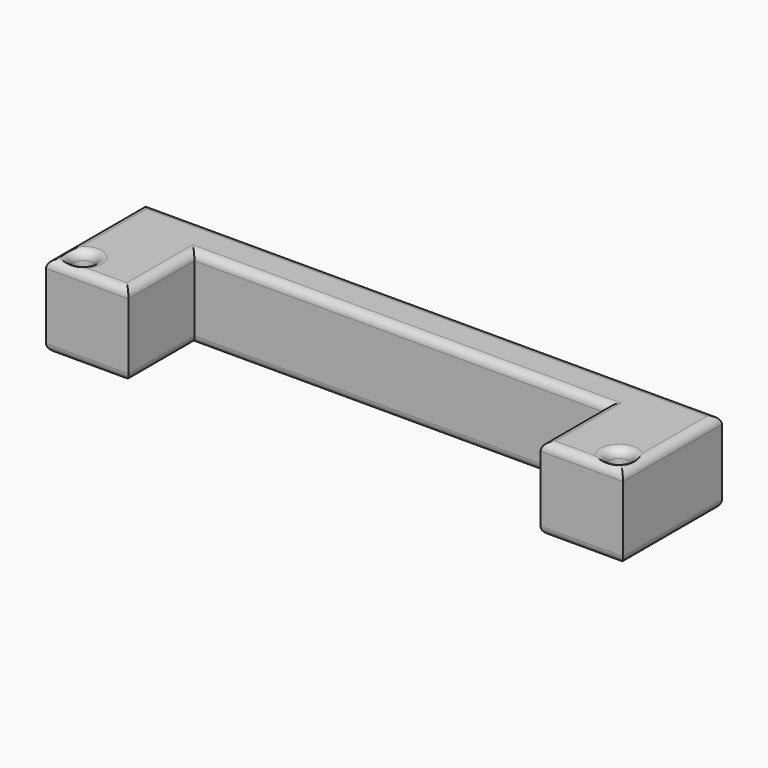
from build123d import *

# Parameters (mm, degrees)
F1_DEPTH     = 20
F3_D         = 5
F5_T1_DEPTH  = 150
F5_T3_DEPTH  = 40
F5_T5_DEPTH  = 30
F5_T7_DEPTH  = 25
F5_T9_DEPTH  = 100
F5_T11_DEPTH = 30
F5_T25_DEPTH = 105
F5_T29_DEPTH = 30
F5_T36_DEPTH = 30
F5_T40_DEPTH = 105
F5_T47_DEPTH = 30
F5_T51_DEPTH = 105
F5_T58_DEPTH = 105
F5_T62_DEPTH = 30


# Not quite as in the source:
# - a fillet or chamfer that OpenCascade refuses, or shapes differently, is made with other operations: its cross-section is extruded or revolved along the edge and cut away or added


with BuildPart() as f1:
    # F0 (on Top) → F1 (new body)
    with BuildSketch(Plane.XY):
        Polygon((70, 30), (0, 30), (0, 20), (50, 20), (50, 0), (70, 0), align=None)
    extrude(amount=F1_DEPTH)

    # F3 (through all)
    with Locations(Plane(origin=(0, 0, 0), x_dir=(1, 0, 0), z_dir=(0, 0, -1))):
        with Locations((65, -5)):
            Hole(F3_D / 2)

    # F4: F1 across plane


with BuildPart() as f1_1:
    add(f1.part)
    add(f1.part.mirror(Plane.YZ))

    # F5: fillet of radius 2 on 20 edges, made by hand

    # F5_s2 → F5_t1 (cut)
    with BuildSketch(Plane.YZ.offset(-75)):
        with BuildLine():
            ThreePointArc((30, 18), (29.4142135624, 19.4142135624), (28, 20))
            Line((28, 20), (30, 20))
            Line((30, 20), (30, 18))
        make_face()
        with BuildLine():
            ThreePointArc((30, 2), (29.4142135624, 0.5857864376), (28, 0))
            Line((28, 0), (30, 0))
            Line((30, 0), (30, 2))
        make_face()
    extrude(amount=F5_T1_DEPTH, mode=Mode.SUBTRACT)

    # F5_s4 → F5_t3 (cut)
    with BuildSketch(Plane.XZ.offset(-35)):
        with BuildLine():
            ThreePointArc((-70, 18), (-69.4142135624, 19.4142135624), (-68, 20))
            Line((-68, 20), (-70, 20))
            Line((-70, 20), (-70, 18))
        make_face()
        with BuildLine():
            ThreePointArc((68, 20), (69.4142135624, 19.4142135624), (70, 18))
            Line((70, 18), (70, 20))
            Line((70, 20), (68, 20))
        make_face()
        with BuildLine():
            ThreePointArc((-68, 0), (-69.4142135624, 0.5857864376), (-70, 2))
            Line((-70, 2), (-70, 0))
            Line((-70, 0), (-68, 0))
        make_face()
        with BuildLine():
            ThreePointArc((68, 0), (69.4142135624, 0.5857864376), (70, 2))
            Line((70, 2), (70, 0))
            Line((70, 0), (68, 0))
        make_face()
    extrude(amount=F5_T3_DEPTH, mode=Mode.SUBTRACT)

    # F5_s6 → F5_t5 (cut)
    with BuildSketch(Plane.YZ.offset(-75)):
        with BuildLine():
            ThreePointArc((0, 18), (0.5857864376, 19.4142135624), (2, 20))
            Line((2, 20), (0, 20))
            Line((0, 20), (0, 18))
        make_face()
        with BuildLine():
            ThreePointArc((2, 0), (0.5857864376, 0.5857864376), (0, 2))
            Line((0, 2), (0, 0))
            Line((0, 0), (2, 0))
        make_face()
    extrude(amount=F5_T5_DEPTH, mode=Mode.SUBTRACT)

    # F5_s8 → F5_t7 (cut)
    with BuildSketch(Plane.XZ.offset(-20)):
        with BuildLine():
            ThreePointArc((-50, 18), (-50.5857864376, 19.4142135624), (-52, 20))
            Line((-52, 20), (-50, 20))
            Line((-50, 20), (-50, 18))
        make_face()
        with BuildLine():
            ThreePointArc((50, 18), (50.5857864376, 19.4142135624), (52, 20))
            Line((52, 20), (50, 20))
            Line((50, 20), (50, 18))
        make_face()
        with BuildLine():
            ThreePointArc((-52, 0), (-50.5857864376, 0.5857864376), (-50, 2))
            Line((-50, 2), (-50, 0))
            Line((-50, 0), (-52, 0))
        make_face()
        with BuildLine():
            ThreePointArc((52, 0), (50.5857864376, 0.5857864376), (50, 2))
            Line((50, 2), (50, 0))
            Line((50, 0), (52, 0))
        make_face()
    extrude(amount=F5_T7_DEPTH, mode=Mode.SUBTRACT)

    # F5_s10 → F5_t9 (cut)
    with BuildSketch(Plane.YZ.offset(-50)):
        with BuildLine():
            ThreePointArc((20, 18), (20.5857864376, 19.4142135624), (22, 20))
            Line((22, 20), (20, 20))
            Line((20, 20), (20, 18))
        make_face()
        with BuildLine():
            ThreePointArc((22, 0), (20.5857864376, 0.5857864376), (20, 2))
            Line((20, 2), (20, 0))
            Line((20, 0), (22, 0))
        make_face()
    extrude(amount=F5_T9_DEPTH, mode=Mode.SUBTRACT)

    # F5_s12 → F5_t11 (cut)
    with BuildSketch(Plane.YZ.offset(45)):
        with BuildLine():
            ThreePointArc((0, 18), (0.5857864376, 19.4142135624), (2, 20))
            Line((2, 20), (0, 20))
            Line((0, 20), (0, 18))
        make_face()
        with BuildLine():
            ThreePointArc((2, 0), (0.5857864376, 0.5857864376), (0, 2))
            Line((0, 2), (0, 0))
            Line((0, 0), (2, 0))
        make_face()
    extrude(amount=F5_T11_DEPTH, mode=Mode.SUBTRACT)

    # F5_s13 → F5_t14 (revolve, cut)
    with BuildSketch(Plane.XZ.offset(-5)):
        with BuildLine():
            ThreePointArc((67.5, 18), (68.0857864376, 19.4142135624), (69.5, 20))
            Line((69.5, 20), (67.5, 20))
            Line((67.5, 20), (67.5, 18))
        make_face()
    revolve(axis=Axis((65, 5, 20), (0, 0, -1)), mode=Mode.SUBTRACT)

    # F5_s15 → F5_t16 (revolve, cut)
    with BuildSketch(Plane.XZ.offset(-5)):
        with BuildLine():
            ThreePointArc((-67.5, 18), (-68.0857864376, 19.4142135624), (-69.5, 20))
            Line((-69.5, 20), (-67.5, 20))
            Line((-67.5, 20), (-67.5, 18))
        make_face()
    revolve(axis=Axis((-65, 5, 20), (0, 0, 1)), mode=Mode.SUBTRACT)

    # F5_s17 → F5_t18 (revolve, cut)
    with BuildSketch(Plane.XZ.offset(-5)):
        with BuildLine():
            ThreePointArc((69.5, 0), (68.0857864376, 0.5857864376), (67.5, 2))
            Line((67.5, 2), (67.5, 0))
            Line((67.5, 0), (69.5, 0))
        make_face()
    revolve(axis=Axis((65, 5, 0), (0, 0, -1)), mode=Mode.SUBTRACT)

    # F5_s19 → F5_t20 (revolve, cut)
    with BuildSketch(Plane.XZ.offset(-5)):
        with BuildLine():
            ThreePointArc((-69.5, 0), (-68.0857864376, 0.5857864376), (-67.5, 2))
            Line((-67.5, 2), (-67.5, 0))
            Line((-67.5, 0), (-69.5, 0))
        make_face()
    revolve(axis=Axis((-65, 5, 0), (0, 0, 1)), mode=Mode.SUBTRACT)


with BuildPart() as f5_tool23:
    # F5_s24 → F5_t25 (new body)
    with BuildSketch(Plane.YZ.offset(-55)):
        with BuildLine():
            ThreePointArc((20, 18), (20.5857864376, 19.4142135624), (22, 20))
            Line((22, 20), (20, 20))
            Line((20, 20), (20, 18))
        make_face()
    extrude(amount=F5_T25_DEPTH)

    split(bisect_by=Plane.YZ.offset(-50), keep=Keep.BOTTOM)


with BuildPart() as f5_tool27:
    # F5_s28 → F5_t29 (new body)
    with BuildSketch(Plane.XZ.offset(-25)):
        with BuildLine():
            ThreePointArc((-50, 18), (-50.5857864376, 19.4142135624), (-52, 20))
            Line((-52, 20), (-50, 20))
            Line((-50, 20), (-50, 18))
        make_face()
    extrude(amount=F5_T29_DEPTH)

    split(bisect_by=Plane.XZ.offset(-20), keep=Keep.BOTTOM)


with BuildPart() as f5_tool23_1:
    add(f5_tool23.part)

    # F5_t31: intersect F5_tool27
    add(f5_tool27.part, mode=Mode.INTERSECT)


with BuildPart() as f1_2:
    add(f1_1.part)

    # F5_t21: cut F5_tool23
    add(f5_tool23_1.part, mode=Mode.SUBTRACT)


with BuildPart() as f5_tool34:
    # F5_s35 → F5_t36 (new body)
    with BuildSketch(Plane.XZ.offset(-25)):
        with BuildLine():
            ThreePointArc((50, 18), (50.5857864376, 19.4142135624), (52, 20))
            Line((52, 20), (50, 20))
            Line((50, 20), (50, 18))
        make_face()
    extrude(amount=F5_T36_DEPTH)

    split(bisect_by=Plane.XZ.offset(-20), keep=Keep.BOTTOM)


with BuildPart() as f5_tool38:
    # F5_s39 → F5_t40 (new body)
    with BuildSketch(Plane.YZ.offset(-50)):
        with BuildLine():
            ThreePointArc((20, 18), (20.5857864376, 19.4142135624), (22, 20))
            Line((22, 20), (20, 20))
            Line((20, 20), (20, 18))
        make_face()
    extrude(amount=F5_T40_DEPTH)

    split(bisect_by=Plane.YZ.offset(50), keep=Keep.TOP)


with BuildPart() as f5_tool34_1:
    add(f5_tool34.part)

    # F5_t42: intersect F5_tool38
    add(f5_tool38.part, mode=Mode.INTERSECT)


with BuildPart() as f1_3:
    add(f1_2.part)

    # F5_t32: cut F5_tool34
    add(f5_tool34_1.part, mode=Mode.SUBTRACT)


with BuildPart() as f5_tool45:
    # F5_s46 → F5_t47 (new body)
    with BuildSketch(Plane.XZ.offset(-25)):
        with BuildLine():
            ThreePointArc((-52, 0), (-50.5857864376, 0.5857864376), (-50, 2))
            Line((-50, 2), (-50, 0))
            Line((-50, 0), (-52, 0))
        make_face()
    extrude(amount=F5_T47_DEPTH)

    split(bisect_by=Plane.XZ.offset(-20), keep=Keep.BOTTOM)


with BuildPart() as f5_tool49:
    # F5_s50 → F5_t51 (new body)
    with BuildSketch(Plane.YZ.offset(50)):
        with BuildLine():
            ThreePointArc((22, 0), (20.5857864376, 0.5857864376), (20, 2))
            Line((20, 2), (20, 0))
            Line((20, 0), (22, 0))
        make_face()
    extrude(amount=-F5_T51_DEPTH)

    split(bisect_by=Plane.YZ.offset(-50), keep=Keep.BOTTOM)


with BuildPart() as f5_tool45_1:
    add(f5_tool45.part)

    # F5_t53: intersect F5_tool49
    add(f5_tool49.part, mode=Mode.INTERSECT)


with BuildPart() as f1_4:
    add(f1_3.part)

    # F5_t43: cut F5_tool45
    add(f5_tool45_1.part, mode=Mode.SUBTRACT)


with BuildPart() as f5_tool56:
    # F5_s57 → F5_t58 (new body)
    with BuildSketch(Plane.YZ.offset(55)):
        with BuildLine():
            ThreePointArc((22, 0), (20.5857864376, 0.5857864376), (20, 2))
            Line((20, 2), (20, 0))
            Line((20, 0), (22, 0))
        make_face()
    extrude(amount=-F5_T58_DEPTH)

    split(bisect_by=Plane.YZ.offset(50), keep=Keep.TOP)


with BuildPart() as f5_tool60:
    # F5_s61 → F5_t62 (new body)
    with BuildSketch(Plane.XZ.offset(-25)):
        with BuildLine():
            ThreePointArc((52, 0), (50.5857864376, 0.5857864376), (50, 2))
            Line((50, 2), (50, 0))
            Line((50, 0), (52, 0))
        make_face()
    extrude(amount=F5_T62_DEPTH)

    split(bisect_by=Plane.XZ.offset(-20), keep=Keep.BOTTOM)


with BuildPart() as f5_tool56_1:
    add(f5_tool56.part)

    # F5_t64: intersect F5_tool60
    add(f5_tool60.part, mode=Mode.INTERSECT)


with BuildPart() as f1_5:
    add(f1_4.part)

    # F5_t54: cut F5_tool56
    add(f5_tool56_1.part, mode=Mode.SUBTRACT)


solid = f1_5.part
